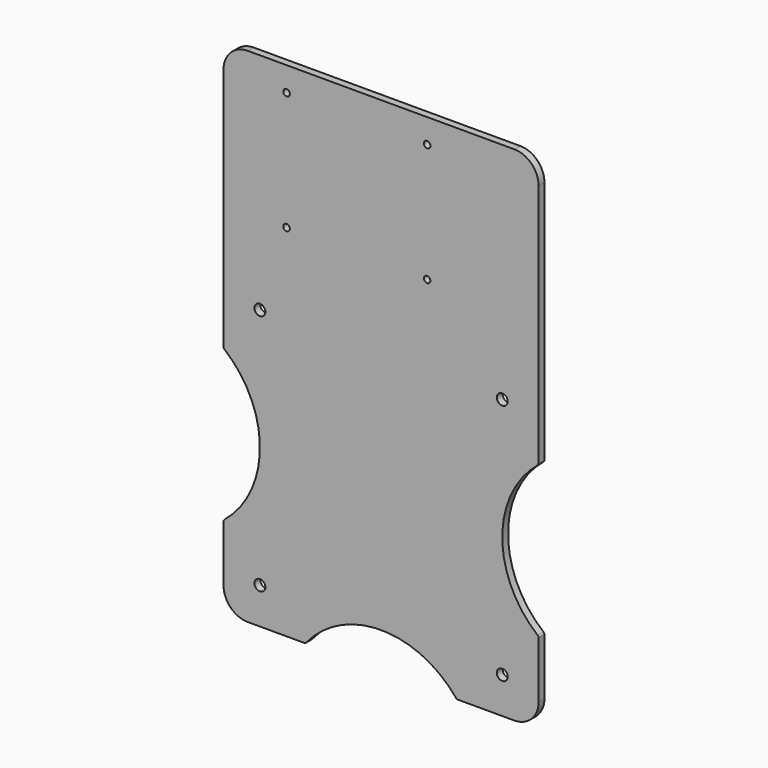
from build123d import *

# Parameters (mm, degrees)
F0_R     = 2.25
F0_R_2   = 1.35
F0_R_3   = 1.3110502125
F1_DEPTH = 3
F2_R     = 1


with BuildPart() as f1:
    # F0 (on Front) → F1 (new body)
    with BuildSketch(Plane.XZ):
        with BuildLine():
            ThreePointArc((0, 10), (2.9289321881, 2.9289321881), (10, 0))
            Line((10, 0), (33.775010008, 0))
            ThreePointArc((33.775010008, 0), (65, 15), (96.224989992, 0))
            Line((96.224989992, 0), (120, 0))
            ThreePointArc((120, 0), (127.0710678119, 2.9289321881), (130, 10))
            Line((130, 10), (130, 33.775010008))
            ThreePointArc((130, 33.775010008), (115, 65), (130, 96.224989992))
            Line((130, 96.224989992), (130, 197.5))
            ThreePointArc((130, 197.5), (127.0710678119, 204.5710678119), (120, 207.5))
            Line((120, 207.5), (10, 207.5))
            ThreePointArc((10, 207.5), (2.9289321881, 204.5710678119), (0, 197.5))
            Line((0, 197.5), (0, 96.224989992))
            ThreePointArc((0, 96.224989992), (15, 65), (0, 33.775010008))
            Line((0, 33.775010008), (0, 10))
        make_face()
        with Locations((15, 15)):
            Circle(F0_R, mode=Mode.SUBTRACT)
        with Locations((115, 15)):
            Circle(F0_R, mode=Mode.SUBTRACT)
        with Locations((15, 115)):
            Circle(F0_R, mode=Mode.SUBTRACT)
        with Locations((26, 148.5)):
            Circle(F0_R_2, mode=Mode.SUBTRACT)
        with Locations((26, 197.5)):
            Circle(F0_R_2, mode=Mode.SUBTRACT)
        with Locations((84, 148.5)):
            Circle(F0_R_3, mode=Mode.SUBTRACT)
        with Locations((115, 115)):
            Circle(F0_R, mode=Mode.SUBTRACT)
        with Locations((84, 197.5)):
            Circle(F0_R_2, mode=Mode.SUBTRACT)
    extrude(amount=F1_DEPTH)

    # F2
    f2_edges = [f1.edges().sort_by_distance(p)[0] for p in [
        (0, -1.5, 33.77501),
        (130, -1.5, 96.22499),
        (33.77501, -1.5, 0),
        (96.22499, -1.5, 0),
        (130, -1.5, 33.77501),
        (0, -1.5, 96.22499),
    ]]
    fillet(f2_edges, radius=F2_R)


solid = f1.part
